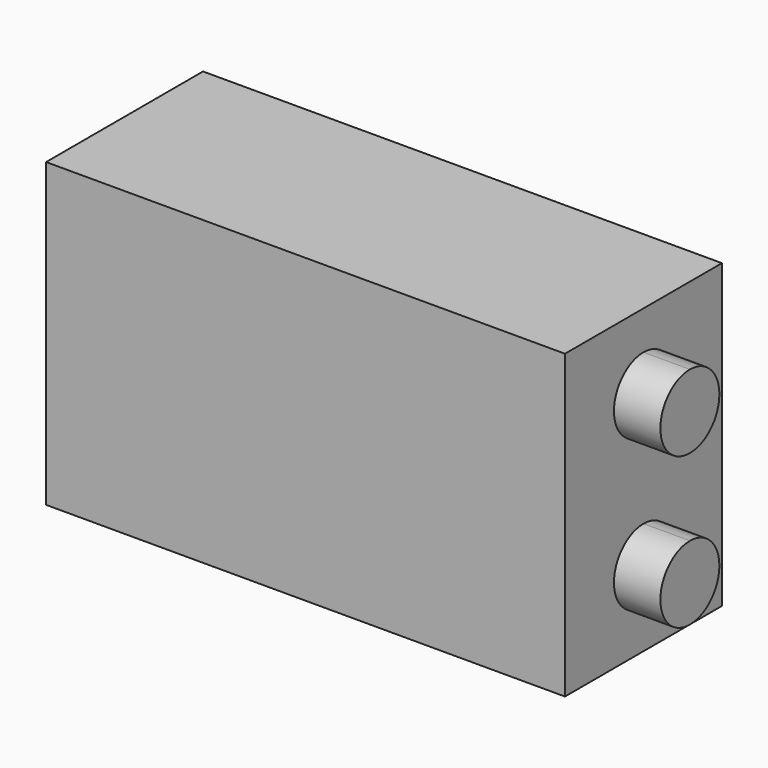
from build123d import *

# Parameters (mm, degrees)
F0_W     = 44.7
F0_H     = 26
F1_DEPTH = 16.9
F3_DEPTH = 4


with BuildPart() as f1:
    # F0 (on Front) → F1 (new body)
    with BuildSketch(Plane.XZ):
        Rectangle(F0_W, F0_H)
    extrude(amount=F1_DEPTH)

    # F2 (on face) → F3 (join)
    with BuildSketch(Plane.YZ.offset(22.35)):
        with BuildLine():
            ThreePointArc((-8.45, -3.325), (-11.625, -6.5), (-8.45, -9.675))
            Line((-8.45, -9.675), (-8.45, -3.325))
        make_face()
        with BuildLine():
            Line((-8.45, -3.325), (-8.45, -9.675))
            ThreePointArc((-8.45, -9.675), (-6.2049359697, -8.7450640303), (-5.275, -6.5))
            ThreePointArc((-5.275, -6.5), (-6.2049359697, -4.2549359697), (-8.45, -3.325))
        make_face()
        with BuildLine():
            ThreePointArc((-8.45, 9.675), (-11.625, 6.5), (-8.45, 3.325))
            Line((-8.45, 3.325), (-8.45, 6.5))
            Line((-8.45, 6.5), (-8.45, 9.675))
        make_face()
        with BuildLine():
            Line((-8.45, 6.5), (-8.45, 3.325))
            ThreePointArc((-8.45, 3.325), (-6.2049359697, 4.2549359697), (-5.275, 6.5))
            ThreePointArc((-5.275, 6.5), (-6.2049359697, 8.7450640303), (-8.45, 9.675))
            Line((-8.45, 9.675), (-8.45, 6.5))
        make_face()
    extrude(amount=F3_DEPTH)


solid = f1.part
